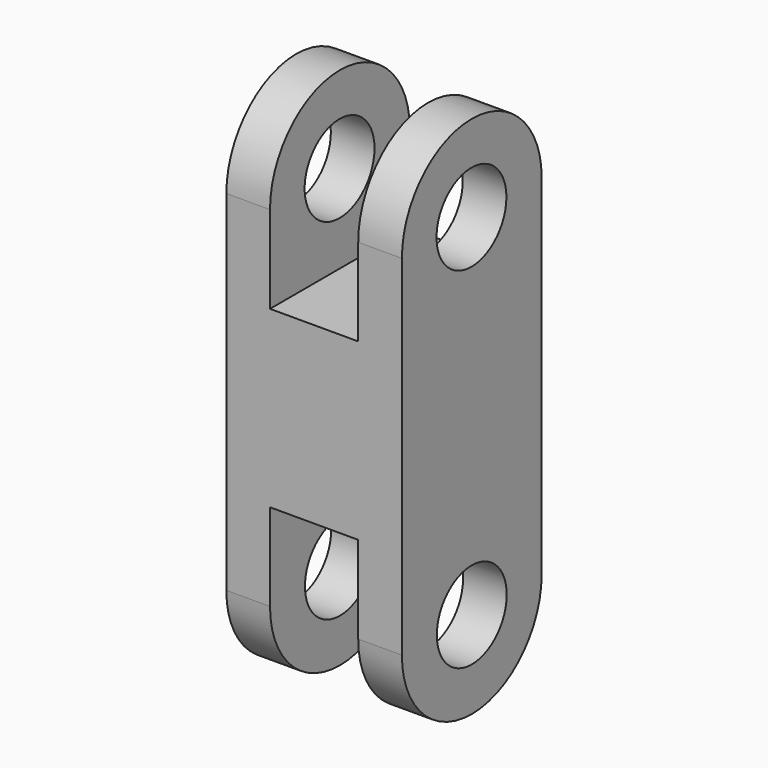
from build123d import *

# Parameters (mm, degrees)
F0_W     = 40
F0_H     = 80
F1_DEPTH = 20.1
F2_R     = 10
F3_DEPTH = 10
F5_W     = 20.2
F5_H     = 40
F6_DEPTH = 20.1
F7_R     = 10
F8_DEPTH = 40.2
F9_R     = 19.99999


# Not quite as in the source:
# - a fillet or chamfer is up to 0.001 mm smaller than in the source, because OpenCascade refuses the exact size


with BuildPart() as f1:
    # F0 (on Right) → F1 (new body)
    with BuildSketch(Plane.YZ):
        Rectangle(F0_W, F0_H)
    extrude(amount=F1_DEPTH)

    # F2 (on face) → F3 (join)
    with BuildSketch(Plane.YZ.offset(20.1)):
        with BuildLine():
            Line((-20, 60), (-20, 40))
            Line((-20, 40), (20, 40))
            Line((20, 40), (20, 60))
            ThreePointArc((20, 60), (0, 80), (-20, 60))
        make_face()
        with Locations((-0.0894565019, 60.1939037442)):
            Circle(F2_R, mode=Mode.SUBTRACT)
    extrude(amount=-F3_DEPTH)

    # F4: F1 across face


with BuildPart() as f1_1:
    add(f1.part)
    add(f1.part.mirror(Plane(origin=(0, 0, 0), x_dir=(0, 1, 0), z_dir=(-1, 0, 0))))

    # F5 (on Front) → F6 (cut, symmetric)
    with BuildSketch(Plane.XZ):
        with Locations((0, -20)):
            Rectangle(F5_W, F5_H)
    extrude(amount=F6_DEPTH, both=True, mode=Mode.SUBTRACT)

    # F7 (on face) → F8 (cut)
    with BuildSketch(Plane.YZ.offset(20.1)):
        with Locations((0, -20)):
            Circle(F7_R)
    extrude(amount=-F8_DEPTH, mode=Mode.SUBTRACT)

    # F9 (radius 20 in the source; OpenCascade refuses exactly that, so slightly less here)
    f9_edges = [f1_1.edges().sort_by_distance(p)[0] for p in [
        (-15.1, -20, -40),
        (15.1, -20, -40),
        (15.1, 20, -40),
        (-15.1, 20, -40),
    ]]
    fillet(f9_edges, radius=F9_R)


solid = f1_1.part
